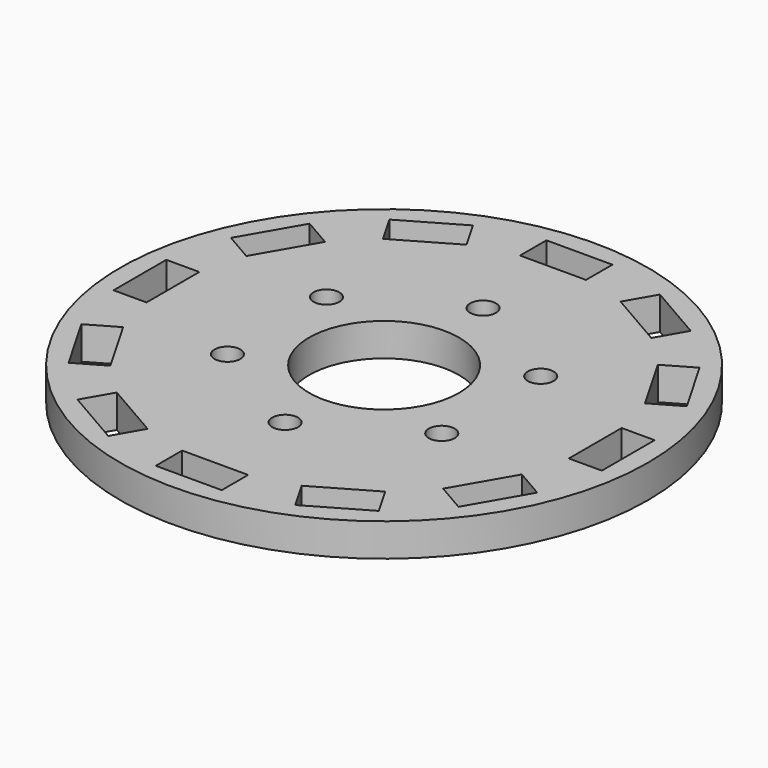
from build123d import *

# Parameters (mm, degrees)
F0_R            = 50.8
F0_R_2          = 14.4272
F1_DEPTH        = 6.35
F2_W            = 12.7
F2_H            = 6.35
F3_DEPTH        = 6.351
F3_COPIES_COUNT = 12
F4_R            = 2.4892
F5_DEPTH        = 6.351
F5_COPIES_COUNT = 6


# Not quite as in the source:
# - a pattern or mirror of a feature is missing from the dataset's text; its kind, count and spacing are read off the source's solid


with BuildPart() as f1:
    # F0 (on Top) → F1 (new body)
    with BuildSketch(Plane.XY):
        Circle(F0_R)
        Circle(F0_R_2, mode=Mode.SUBTRACT)
    extrude(amount=F1_DEPTH)

    # F2 (on face) → F3 (cut, through all)
    with BuildSketch(Plane.XY.offset(6.35)):
        with Locations((0, 43.815)):
            Rectangle(F2_W, F2_H)
    f3 = extrude(amount=-F3_DEPTH, mode=Mode.SUBTRACT)

    # F3_copies: F3 ×12 about axis
    f3_copies_axis = Axis((0, 0, 0), (0, 0, 1))
    for i in range(1, F3_COPIES_COUNT):
        add(f3.rotate(f3_copies_axis, i * 360 / F3_COPIES_COUNT), mode=Mode.SUBTRACT)

    # F4 (on face) → F5 (cut, through all)
    with BuildSketch(Plane.XY.offset(6.35)):
        with Locations((0, 23.8125)):
            Circle(F4_R)
    f5 = extrude(amount=-F5_DEPTH, mode=Mode.SUBTRACT)

    # F5_copies: F5 ×6 about axis
    f5_copies_axis = Axis((0, 0, 0), (0, 0, 1))
    for i in range(1, F5_COPIES_COUNT):
        add(f5.rotate(f5_copies_axis, i * 360 / F5_COPIES_COUNT), mode=Mode.SUBTRACT)


solid = f1.part
